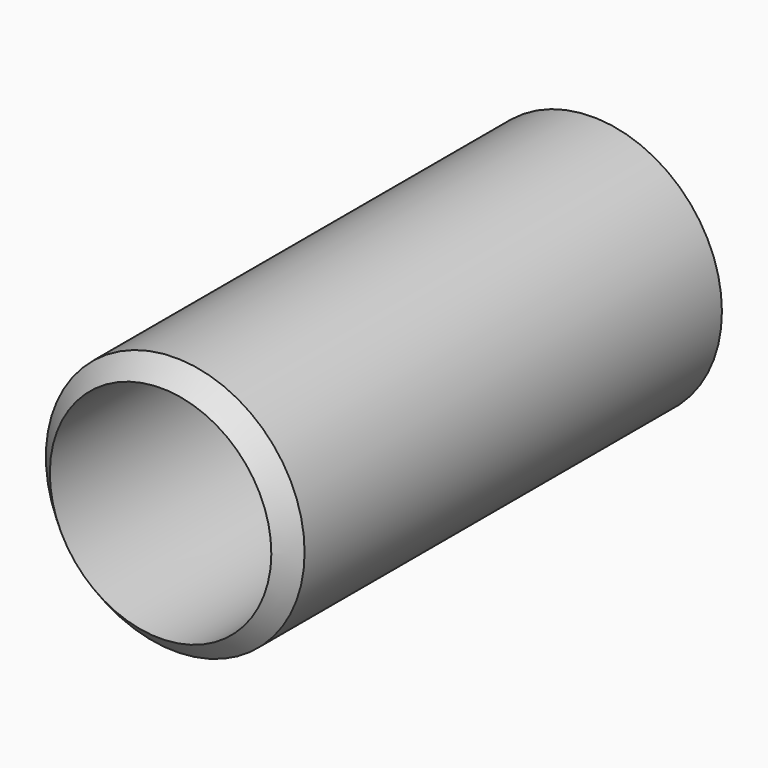
from build123d import *

# Parameters (mm, degrees)
F0_R     = 35.2770555377
F0_R_2   = 30.0400114969
F1_DEPTH = 152.4


# Not quite as in the source:
# - a fillet or chamfer that OpenCascade refuses, or shapes differently, is made with other operations: its cross-section is extruded or revolved along the edge and cut away or added


with BuildPart() as f1:
    # F0 (on Front) → F1 (new body)
    with BuildSketch(Plane.XZ):
        Circle(F0_R)
        with Locations((0.1925629913, 0.0962815902)):
            Circle(F0_R_2, mode=Mode.SUBTRACT)
    extrude(amount=F1_DEPTH)

    # F2: chamfer of 10.16 on 1 edges, made by hand

    # F2_s1 → F2_t2 (revolve, cut)
    with BuildSketch(Plane.XY):
        Polygon((35.2770555377, -142.24), (25.1170555377, -152.4), (35.2770555377, -152.4), align=None)
    revolve(axis=Axis((0, -152.4, 0), (0, -1, 0)), mode=Mode.SUBTRACT)


solid = f1.part
